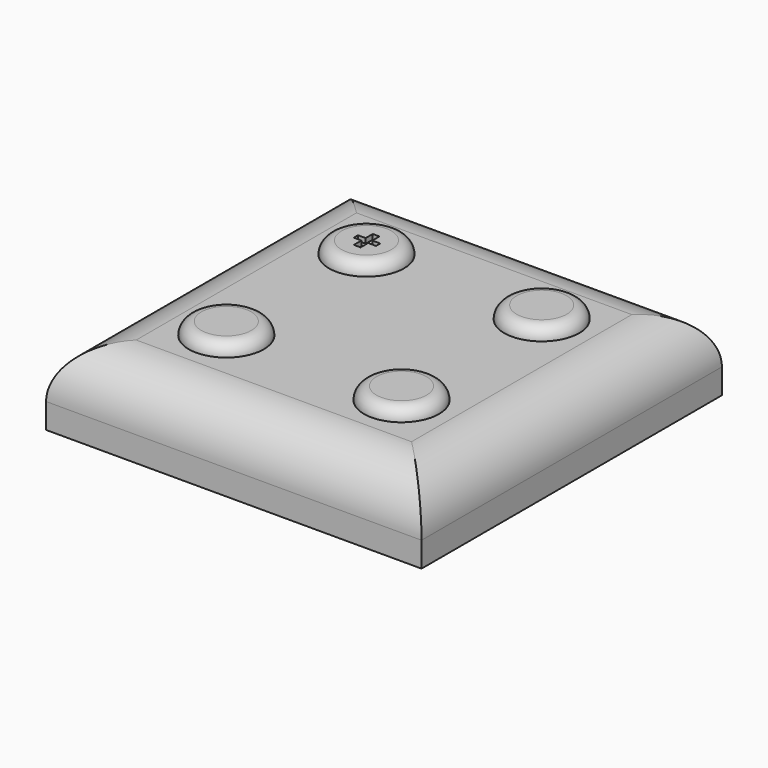
from build123d import *

# Parameters (mm, degrees)
F0_W     = 38.1
F0_H     = 38.1
F1_DEPTH = 7.62
F2_R     = 5.08
F3_R     = 3.81
F4_DEPTH = 1.27
F5_R     = 1.26999
F5_2_R   = 1.26999
F5_3_R   = 1.26999
F5_4_R   = 1.26999
F6_W     = 0.684382394
F6_H     = 0.8962163702
F6_W_2   = 0.7821517065
F6_H_2   = 0.5377288908
F6_W_3   = 0.7984461263
F6_H_3   = 0.9613940492
F7_DEPTH = 0.508


# Not quite as in the source:
# - a fillet or chamfer is up to 0.001 mm smaller than in the source, because OpenCascade refuses the exact size
# - a feature of the source that left no trace in its solid (it failed there, or was rolled back) is left out


with BuildPart() as f1:
    # F0 (on Top) → F1 (new body)
    with BuildSketch(Plane.XY):
        Rectangle(F0_W, F0_H)
    extrude(amount=F1_DEPTH)

    # F2
    f2_edges = [f1.edges().sort_by_distance(p)[0] for p in [
        (-19.05, 0, 7.62),
        (0, 19.05, 7.62),
        (19.05, 0, 7.62),
        (0, -19.05, 7.62),
    ]]
    fillet(f2_edges, radius=F2_R)


with BuildPart() as f4:
    # F3 (on face) → F4 (new body)
    with BuildSketch(Plane.XY.offset(7.62)):
        with Locations((8.89, 8.89)):
            Circle(F3_R)
    extrude(amount=F4_DEPTH)

    # F5 (radius 1.27 in the source; OpenCascade refuses exactly that, so slightly less here)
    f5_edges = [f4.edges().sort_by_distance(p)[0] for p in [
        (5.08, 8.89, 8.89),
    ]]
    fillet(f5_edges, radius=F5_R)


with BuildPart() as f4b:
    # F3 (on face) → F4, piece 2 (new body)
    with BuildSketch(Plane.XY.offset(7.62)):
        with Locations((8.89, -8.89)):
            Circle(F3_R)
    extrude(amount=F4_DEPTH)

    # F5#2 (radius 1.27 in the source; OpenCascade refuses exactly that, so slightly less here)
    f5_2_edges = [f4b.edges().sort_by_distance(p)[0] for p in [
        (5.08, -8.89, 8.89),
    ]]
    fillet(f5_2_edges, radius=F5_2_R)


with BuildPart() as f4c:
    # F3 (on face) → F4, piece 3 (new body)
    with BuildSketch(Plane.XY.offset(7.62)):
        with Locations((-8.89, -8.89)):
            Circle(F3_R)
    extrude(amount=F4_DEPTH)

    # F5#3 (radius 1.27 in the source; OpenCascade refuses exactly that, so slightly less here)
    f5_3_edges = [f4c.edges().sort_by_distance(p)[0] for p in [
        (-12.7, -8.89, 8.89),
    ]]
    fillet(f5_3_edges, radius=F5_3_R)


with BuildPart() as f4d:
    # F3 (on face) → F4, piece 4 (new body)
    with BuildSketch(Plane.XY.offset(7.62)):
        with Locations((-8.89, 8.89)):
            Circle(F3_R)
    extrude(amount=F4_DEPTH)

    # F5#4 (radius 1.27 in the source; OpenCascade refuses exactly that, so slightly less here)
    f5_4_edges = [f4d.edges().sort_by_distance(p)[0] for p in [
        (-12.7, 8.89, 8.89),
    ]]
    fillet(f5_4_edges, radius=F5_4_R)

    # F6 (on face) → F7 (cut)
    with BuildSketch(Plane.XY.offset(8.89)):
        with Locations((-8.8372193277, 9.5931137912)):
            Rectangle(F6_W, F6_H)
        with Locations((-9.5704863779, 8.8761411607)):
            Rectangle(F6_W_2, F6_H_2)
        with Locations((-8.8372193277, 8.8761411607)):
            Rectangle(F6_W, F6_H_2)
        with Locations((-8.0958050676, 8.8761411607)):
            Rectangle(F6_W_3, F6_H_2)
        with Locations((-8.8372193277, 8.1265796907)):
            Rectangle(F6_W, F6_H_3)
        with Locations((8.8355047628, 8.2747801207)):
            Rectangle(F6_W, F6_H_3)
        with Locations((8.1022377126, 9.0243415907)):
            Rectangle(F6_W_2, F6_H_2)
        with Locations((8.8355047628, 9.0243415907)):
            Rectangle(F6_W, F6_H_2)
        with Locations((8.8355047628, 9.7413142212)):
            Rectangle(F6_W, F6_H)
        with Locations((9.5769190229, 9.0243415907)):
            Rectangle(F6_W_3, F6_H_2)
        with Locations((-9.6729216166, -8.7657244876)):
            Rectangle(F6_W_2, F6_H_2)
        with Locations((-8.9396545663, -8.7657244876)):
            Rectangle(F6_W, F6_H_2)
        with Locations((-8.9396545663, -8.0487518571)):
            Rectangle(F6_W, F6_H)
        with Locations((-8.1982403062, -8.7657244876)):
            Rectangle(F6_W_3, F6_H_2)
        with Locations((8.8686496019, -9.6509321593)):
            Rectangle(F6_W, F6_H_3)
        with Locations((8.1353825517, -8.9013706893)):
            Rectangle(F6_W_2, F6_H_2)
        with Locations((9.6100638621, -8.9013706893)):
            Rectangle(F6_W_3, F6_H_2)
        with Locations((8.8686496019, -8.1843980588)):
            Rectangle(F6_W, F6_H)
        with Locations((8.8686496019, -8.9013706893)):
            Rectangle(F6_W, F6_H_2)
        with Locations((-8.9396545663, -9.5152859576)):
            Rectangle(F6_W, F6_H_3)
    extrude(amount=-F7_DEPTH, mode=Mode.SUBTRACT)


solid = Compound([f1.part, f4.part, f4b.part, f4c.part, f4d.part])
